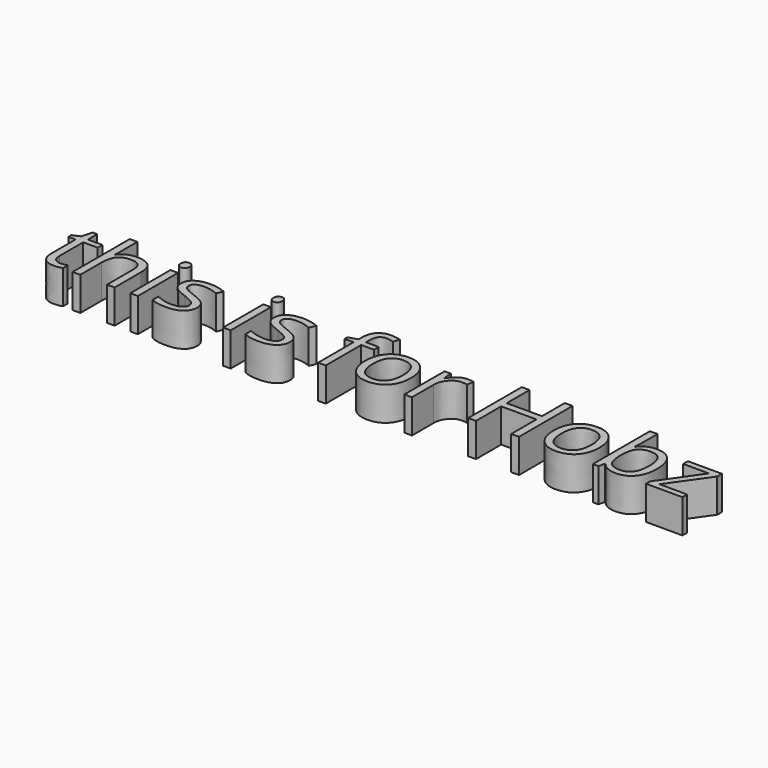
from build123d import *

# Parameters (mm, degrees)
F0_TEXT_SIZE = 70.7342703309
F1_DEPTH     = 25.4


# Not quite as in the source:
# - Text() gives the source's letters only with a copy of the font that has no kerning and outlines rounded to 1/6400 em; it was checked with that copy


with BuildPart() as f1:
    # F0 (on Top) → F1 (new body)
    with BuildSketch(Plane.XY):
        with Locations((-50.9388148785, -34.2350490391)):
            Text('this is for Hobz', F0_TEXT_SIZE, font='Open Sans', text_align=(TextAlign.LEFT, TextAlign.BOTTOM))
    extrude(amount=F1_DEPTH)


solid = f1.part
